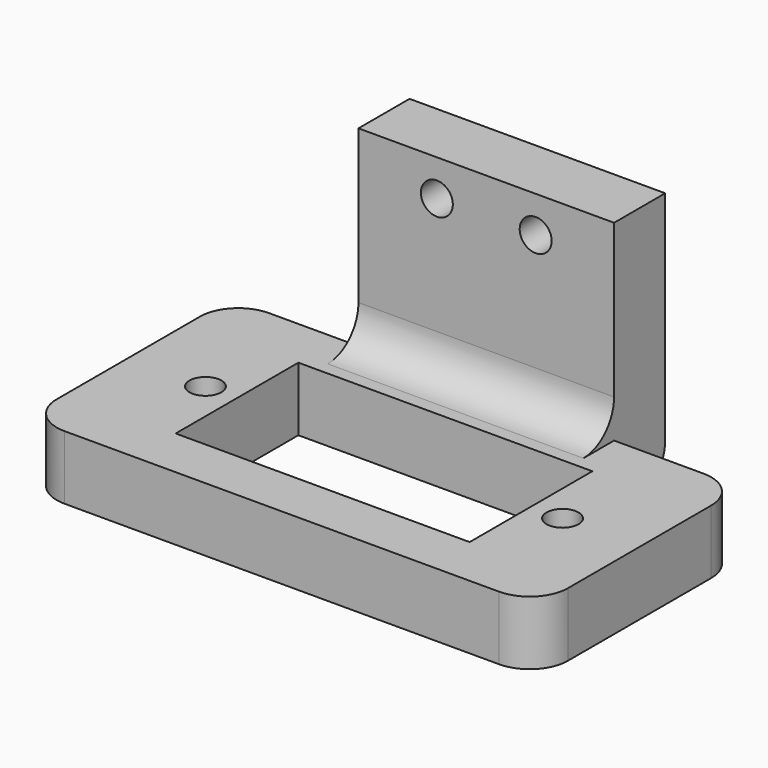
from build123d import *

# Parameters (mm, degrees)
F1_DEPTH    = 20
F0_R        = 1.25
F0_W        = 23
F0_H        = 12
F2_DEPTH    = 5
F3_R        = 1.25
F4_DEPTH    = 5
F5_T1_DEPTH = 20
F5_T3_DEPTH = 20
F5_T5_DEPTH = 35


# Not quite as in the source:
# - a fillet or chamfer that OpenCascade refuses, or shapes differently, is made with other operations: its cross-section is extruded or revolved along the edge and cut away or added


with BuildPart() as f1:
    # F0 (on Top) → F1 (new body)
    with BuildSketch(Plane.XY):
        Polygon((-10, 15), (-10, 10), (10, 10), (10, 15), (0, 15), align=None)
    extrude(amount=F1_DEPTH)

    # F0 (on Top) → F2 (join)
    with BuildSketch(Plane.XY):
        Polygon((-10, 10), (-20, 10), (-20, -10), (20, -10), (20, 10), (10, 10), align=None)
        with Locations((-13.97, 0)):
            Circle(F0_R, mode=Mode.SUBTRACT)
        Rectangle(F0_W, F0_H, mode=Mode.SUBTRACT)
        with Locations((13.97, 0)):
            Circle(F0_R, mode=Mode.SUBTRACT)
    extrude(amount=F2_DEPTH)

    # F3 (on face) → F4 (cut)
    with BuildSketch(Plane(origin=(0, 15, 0), x_dir=(-1, 0, 0), z_dir=(0, 1, 0))):
        with Locations((3.865, 17.1576076342)):
            Circle(F3_R)
        with Locations((-3.865, 17.1576076342)):
            Circle(F3_R)
    extrude(amount=-F4_DEPTH, mode=Mode.SUBTRACT)

    # F5: fillet of radius 3 on 8 edges, made by hand

    # F5_s2 → F5_t1 (join)
    with BuildSketch(Plane.YZ.offset(-10)):
        with BuildLine():
            ThreePointArc((10, 8), (9.1213203436, 5.8786796564), (7, 5))
            Line((7, 5), (10, 5))
            Line((10, 5), (10, 8))
        make_face()
    extrude(amount=F5_T1_DEPTH)

    # F5_s4 → F5_t3 (cut)
    with BuildSketch(Plane.XY.offset(-7.5)):
        with BuildLine():
            ThreePointArc((-17, 10), (-19.1213203436, 9.1213203436), (-20, 7))
            Line((-20, 7), (-20, 10))
            Line((-20, 10), (-17, 10))
        make_face()
        with BuildLine():
            ThreePointArc((20, 7), (19.1213203436, 9.1213203436), (17, 10))
            Line((17, 10), (20, 10))
            Line((20, 10), (20, 7))
        make_face()
        with BuildLine():
            ThreePointArc((17, -10), (19.1213203436, -9.1213203436), (20, -7))
            Line((20, -7), (20, -10))
            Line((20, -10), (17, -10))
        make_face()
        with BuildLine():
            ThreePointArc((-20, -7), (-19.1213203436, -9.1213203436), (-17, -10))
            Line((-17, -10), (-20, -10))
            Line((-20, -10), (-20, -7))
        make_face()
    extrude(amount=F5_T3_DEPTH, mode=Mode.SUBTRACT)

    # F5_s6 → F5_t5 (cut)
    with BuildSketch(Plane.YZ.offset(-17.5)):
        with BuildLine():
            ThreePointArc((15, 3), (14.1213203436, 0.8786796564), (12, 0))
            Line((12, 0), (15, 0))
            Line((15, 0), (15, 3))
        make_face()
    extrude(amount=F5_T5_DEPTH, mode=Mode.SUBTRACT)


solid = f1.part
